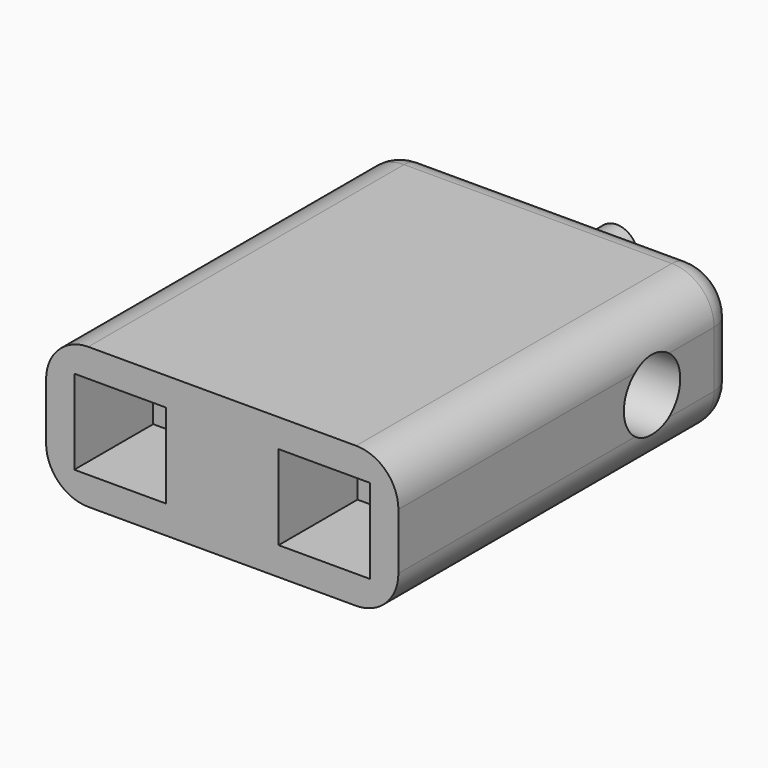
from build123d import *

# Parameters (mm, degrees)
F0_W         = 25
F0_H         = 30
F1_DEPTH     = 10
F2_R         = 1.5
F3_DEPTH     = 5
F4_R         = 2.5
F5_DEPTH     = 5
F6_R         = 2.5
F7_DEPTH     = 5
F8_W         = 6.5
F8_H         = 6
F9_DEPTH     = 7
F10_T1_DEPTH = 45
F11_R        = 2


# Not quite as in the source:
# - a fillet or chamfer that OpenCascade refuses, or shapes differently, is made with other operations: its cross-section is extruded or revolved along the edge and cut away or added


with BuildPart() as f1:
    # F0 (on Top) → F1 (new body)
    with BuildSketch(Plane.XY):
        Rectangle(F0_W, F0_H)
    extrude(amount=F1_DEPTH)

    # F2 (on face) → F3 (join)
    with BuildSketch(Plane(origin=(0, 15, 0), x_dir=(-1, 0, 0), z_dir=(0, 1, 0))):
        with Locations((0, 5)):
            Circle(F2_R)
    extrude(amount=F3_DEPTH)

    # F4 (on face) → F5 (cut)
    with BuildSketch(Plane.YZ.offset(12.5)):
        with Locations((7.5, 5)):
            Circle(F4_R)
    extrude(amount=-F5_DEPTH, mode=Mode.SUBTRACT)

    # F6 (on face) → F7 (cut)
    with BuildSketch(Plane(origin=(-12.5, 0, 0), x_dir=(0, -1, 0), z_dir=(-1, 0, 0))):
        with Locations((-7.5, 5)):
            Circle(F6_R)
    extrude(amount=-F7_DEPTH, mode=Mode.SUBTRACT)

    # F8 (on face) → F9 (cut)
    with BuildSketch(Plane.XZ.offset(15)):
        with Locations((7.25, 5)):
            Rectangle(F8_W, F8_H)
        with Locations((-7.25, 5)):
            Rectangle(F8_W, F8_H)
    extrude(amount=-F9_DEPTH, mode=Mode.SUBTRACT)

    # F10: fillet of radius 3 on 4 edges, made by hand

    # F10_s2 → F10_t1 (cut)
    with BuildSketch(Plane.XZ.offset(-22.5)):
        with BuildLine():
            ThreePointArc((-9.5, 10), (-11.6213203436, 9.1213203436), (-12.5, 7))
            Line((-12.5, 7), (-12.5, 10))
            Line((-12.5, 10), (-9.5, 10))
        make_face()
        with BuildLine():
            ThreePointArc((12.5, 7), (11.6213203436, 9.1213203436), (9.5, 10))
            Line((9.5, 10), (12.5, 10))
            Line((12.5, 10), (12.5, 7))
        make_face()
        with BuildLine():
            ThreePointArc((12.5, 3), (11.6213203436, 0.8786796564), (9.5, 0))
            Line((9.5, 0), (12.5, 0))
            Line((12.5, 0), (12.5, 3))
        make_face()
        with BuildLine():
            ThreePointArc((-9.5, 0), (-11.6213203436, 0.8786796564), (-12.5, 3))
            Line((-12.5, 3), (-12.5, 0))
            Line((-12.5, 0), (-9.5, 0))
        make_face()
    extrude(amount=F10_T1_DEPTH, mode=Mode.SUBTRACT)

    # F11
    f11_edges = [f1.edges().sort_by_distance(p)[0] for p in [
        (11.62132, 15, 0.87868),
        (12.5, 15, 5),
        (11.62132, 15, 9.12132),
        (0, 15, 0),
        (-11.62132, 15, 0.87868),
        (-12.5, 15, 5),
        (-11.62132, 15, 9.12132),
        (0, 15, 10),
    ]]
    fillet(f11_edges, radius=F11_R)


solid = f1.part
